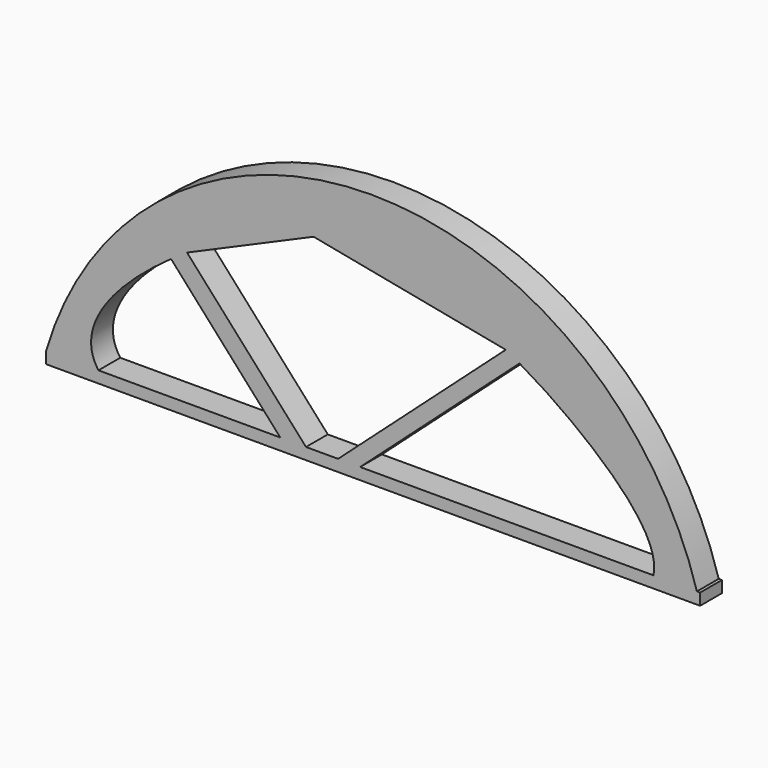
from build123d import *

# Parameters (mm, degrees)
F1_DEPTH = 76.2


with BuildPart() as f1:
    # F0 (on Front) → F1 (new body)
    with BuildSketch(Plane.XZ):
        with BuildLine():
            Line((900.6498717056, -312.5507702395), (891.7103917568, -312.5507702395))
            ThreePointArc((891.7103917568, -312.5507702395), (-18.2198682688, 368.2339185386), (-928.1501282944, -312.5507702395))
            Line((-928.1501282944, -312.5507702395), (-928.1501282944, -345.05851352))
            Line((-928.1501282944, -345.05851352), (-749.2538985146, -345.05851352))
            add(Edge.make_bspline(
                [(-749.2538985146, -345.0585135201), (-760.7342074403, -336.2080146902), (-770.4190479747, -326.955384148), (-778.1336966335, -317.3006312947)],
                knots=[0.9863041687, 0.9863041687, 0.9863041687, 0.9863041687, 1, 1, 1, 1], degree=3))
            add(Edge.make_bspline(
                [(-778.1336966335, -317.3006312947), (-779.3903781429, -315.7279155528), (-780.5947807249, -314.1445295186), (-781.7476175602, -312.5507702395)],
                knots=[0, 0, 0, 0, 0.0022309892, 0.0022309892, 0.0022309892, 0.0022309892], degree=3))
            add(Edge.make_bspline(
                [(-781.7476175602, -312.5507702395), (-852.1024790666, -215.2874716318), (-730.4075461351, -79.390396257), (-578.7611195863, 27.6247892302)],
                knots=[0.0022309892, 0.0022309892, 0.0022309892, 0.0022309892, 0.1383828997, 0.1383828997, 0.1383828997, 0.1383828997], degree=3))
            add(Edge.make_bspline(
                [(-578.7611195863, 27.6247892302), (-564.0565616619, 38.0016311354), (-549.0703872563, 48.1069134214), (-533.9503839152, 57.8790810031)],
                knots=[0.1383828997, 0.1383828997, 0.1383828997, 0.1383828997, 0.1515850153, 0.1515850153, 0.1515850153, 0.1515850153], degree=3))
            add(Edge.make_bspline(
                [(-533.9503839241, 57.8790809984), (-602.4722852405, 100.7350307252), (-409.6251199582, 190.8667602879), (-180.120050854, 211.9691197295)],
                knots=[0, 0, 0, 0, 0.2694339971, 0.2694339971, 0.2694339971, 0.2694339971], degree=3))
            add(Edge.make_bspline(
                [(-180.1200508538, 211.9691197281), (-93.8173354063, 228.6015651353), (-14.6508277799, 226.1155115237), (65.4117966901, 211.4804253565)],
                knots=[0.2631178936, 0.2631178936, 0.2631178936, 0.2631178936, 0.3555862093, 0.3555862093, 0.3555862093, 0.3555862093], degree=3))
            add(Edge.make_bspline(
                [(65.4117966901, 211.4804253565), (252.144781627, 195.4027277771), (400.2346102312, 147.7404794914), (357.158674228, 108.3680934352)],
                knots=[0.3646274658, 0.3646274658, 0.3646274658, 0.3646274658, 0.5902554086, 0.5902554086, 0.5902554086, 0.5902554086], degree=3))
            add(Edge.make_bspline(
                [(357.1586742266, 108.3680934339), (369.9420280531, 101.672338017), (382.7382890401, 94.6802256262), (395.5442289819, 87.3893097061)],
                knots=[0.4659511905, 0.4659511905, 0.4659511905, 0.4659511905, 0.4802734469, 0.4802734469, 0.4802734469, 0.4802734469], degree=3))
            add(Edge.make_bspline(
                [(395.5442289819, 87.3893097061), (452.0964892557, 55.1919250067), (621.2097193886, -58.1382004272), (789.5300294959, -225.1035077486), (769.7574939756, -312.5507702395)],
                knots=[0.4802734469, 0.4802734469, 0.4802734469, 0.4802734469, 0.5435219059, 0.668781717, 0.668781717, 0.668781717, 0.668781717], degree=3))
            add(Edge.make_bspline(
                [(769.7574939756, -312.5507702395), (767.2117421615, -323.809772753), (762.4841536184, -334.6792525956), (755.294559917, -345.05851352)],
                knots=[0.668781717, 0.668781717, 0.668781717, 0.668781717, 0.6849091576, 0.6849091576, 0.6849091576, 0.6849091576], degree=3))
            Line((755.2945599171, -345.05851352), (900.6498717056, -345.05851352))
            Line((900.6498717056, -345.05851352), (900.6498717056, -312.5507702395))
        make_face()
        with BuildLine():
            add(Edge.make_bspline(
                [(-749.2538985146, -345.0585135201), (-760.7342074403, -336.2080146902), (-770.4190479747, -326.955384148), (-778.1336966335, -317.3006312947)],
                knots=[0.9863041687, 0.9863041687, 0.9863041687, 0.9863041687, 1, 1, 1, 1], degree=3))
            Line((-749.2538985146, -345.05851352), (755.2945599171, -345.05851352))
            add(Edge.make_bspline(
                [(769.7574939756, -312.5507702395), (767.2117421615, -323.809772753), (762.4841536184, -334.6792525956), (755.294559917, -345.05851352)],
                knots=[0.668781717, 0.668781717, 0.668781717, 0.668781717, 0.6849091576, 0.6849091576, 0.6849091576, 0.6849091576], degree=3))
            Line((769.7574939756, -312.5507702395), (-49.9293302995, -312.5507702395))
            Line((-49.9293302995, -312.5507702395), (395.5442289819, 87.3893097061))
            add(Edge.make_bspline(
                [(357.1586742266, 108.3680934339), (369.9420280531, 101.672338017), (382.7382890401, 94.6802256262), (395.5442289819, 87.3893097061)],
                knots=[0.4659511905, 0.4659511905, 0.4659511905, 0.4659511905, 0.4802734469, 0.4802734469, 0.4802734469, 0.4802734469], degree=3))
            add(Edge.make_bspline(
                [(357.158674228, 108.3680934352), (356.9910150595, 108.2148491387), (356.8204599128, 108.0617304257), (356.6470209458, 107.9087381034)],
                knots=[0.5902554086, 0.5902554086, 0.5902554086, 0.5902554086, 0.5911335925, 0.5911335925, 0.5911335925, 0.5911335925], degree=3))
            Line((356.6470209458, 107.9087381034), (-111.6821191112, -312.5507702395))
            Line((-111.6821191112, -312.5507702395), (-201.3835205481, -312.5507702395))
            Line((-201.3835205481, -312.5507702395), (-533.9503839109, 57.8790810059))
            add(Edge.make_bspline(
                [(-578.7611195863, 27.6247892302), (-564.0565616619, 38.0016311354), (-549.0703872563, 48.1069134214), (-533.9503839152, 57.8790810031)],
                knots=[0.1383828997, 0.1383828997, 0.1383828997, 0.1383828997, 0.1515850153, 0.1515850153, 0.1515850153, 0.1515850153], degree=3))
            Line((-578.7611195863, 27.6247892302), (-273.35614635, -312.5507702395))
            Line((-273.35614635, -312.5507702395), (-781.7476175602, -312.5507702395))
            add(Edge.make_bspline(
                [(-778.1336966335, -317.3006312947), (-779.3903781429, -315.7279155528), (-780.5947807249, -314.1445295186), (-781.7476175602, -312.5507702395)],
                knots=[0, 0, 0, 0, 0.0022309892, 0.0022309892, 0.0022309892, 0.0022309892], degree=3))
        make_face()
        with BuildLine():
            Line((-180.120050854, 211.9691197295), (357.1586742266, 108.3680934339))
            add(Edge.make_bspline(
                [(65.4117966901, 211.4804253565), (71.5175240267, 210.3643259746), (167.1573362354, 191.7908820713), (264.946329488, 156.6677270957), (357.1586742266, 108.3680934339)],
                knots=[0.3555862093, 0.3555862093, 0.3555862093, 0.3555862093, 0.3626380181, 0.4659511905, 0.4659511905, 0.4659511905, 0.4659511905], degree=3))
            add(Edge.make_bspline(
                [(-180.120050854, 211.9691197295), (-99.0338336855, 219.424774226), (-13.3717100026, 218.2636800411), (65.4117966901, 211.4804253565)],
                knots=[0.2694339971, 0.2694339971, 0.2694339971, 0.2694339971, 0.3646274658, 0.3646274658, 0.3646274658, 0.3646274658], degree=3))
        make_face()
        with BuildLine():
            add(Edge.make_bspline(
                [(65.4117966901, 211.4804253565), (71.5175240267, 210.3643259746), (167.1573362354, 191.7908820713), (264.946329488, 156.6677270957), (357.1586742266, 108.3680934339)],
                knots=[0.3555862093, 0.3555862093, 0.3555862093, 0.3555862093, 0.3626380181, 0.4659511905, 0.4659511905, 0.4659511905, 0.4659511905], degree=3))
            add(Edge.make_bspline(
                [(65.4117966901, 211.4804253565), (252.144781627, 195.4027277771), (400.2346102312, 147.7404794914), (357.158674228, 108.3680934352)],
                knots=[0.3646274658, 0.3646274658, 0.3646274658, 0.3646274658, 0.5902554086, 0.5902554086, 0.5902554086, 0.5902554086], degree=3))
        make_face()
        with BuildLine():
            add(Edge.make_bspline(
                [(-533.9503839241, 57.8790809984), (-602.4722852405, 100.7350307252), (-409.6251199582, 190.8667602879), (-180.120050854, 211.9691197295)],
                knots=[0, 0, 0, 0, 0.2694339971, 0.2694339971, 0.2694339971, 0.2694339971], degree=3))
            add(Edge.make_bspline(
                [(-533.9503839152, 57.8790810031), (-491.8326282353, 85.1000913023), (-360.9478670377, 159.8172978773), (-249.892894391, 198.5223468773), (-180.1200508538, 211.9691197281)],
                knots=[0.1515850153, 0.1515850153, 0.1515850153, 0.1515850153, 0.1883603696, 0.2631178936, 0.2631178936, 0.2631178936, 0.2631178936], degree=3))
        make_face()
        with BuildLine():
            add(Edge.make_bspline(
                [(-533.9503839152, 57.8790810031), (-491.8326282353, 85.1000913023), (-360.9478670377, 159.8172978773), (-249.892894391, 198.5223468773), (-180.1200508538, 211.9691197281)],
                knots=[0.1515850153, 0.1515850153, 0.1515850153, 0.1515850153, 0.1883603696, 0.2631178936, 0.2631178936, 0.2631178936, 0.2631178936], degree=3))
            Line((-533.9503839109, 57.8790810059), (-180.120050854, 211.9691197295))
        make_face()
        with BuildLine():
            add(Edge.make_bspline(
                [(-180.120050854, 211.9691197295), (-99.0338336855, 219.424774226), (-13.3717100026, 218.2636800411), (65.4117966901, 211.4804253565)],
                knots=[0.2694339971, 0.2694339971, 0.2694339971, 0.2694339971, 0.3646274658, 0.3646274658, 0.3646274658, 0.3646274658], degree=3))
            add(Edge.make_bspline(
                [(-180.1200508538, 211.9691197281), (-93.8173354063, 228.6015651353), (-14.6508277799, 226.1155115237), (65.4117966901, 211.4804253565)],
                knots=[0.2631178936, 0.2631178936, 0.2631178936, 0.2631178936, 0.3555862093, 0.3555862093, 0.3555862093, 0.3555862093], degree=3))
        make_face()
    extrude(amount=F1_DEPTH)


solid = f1.part
